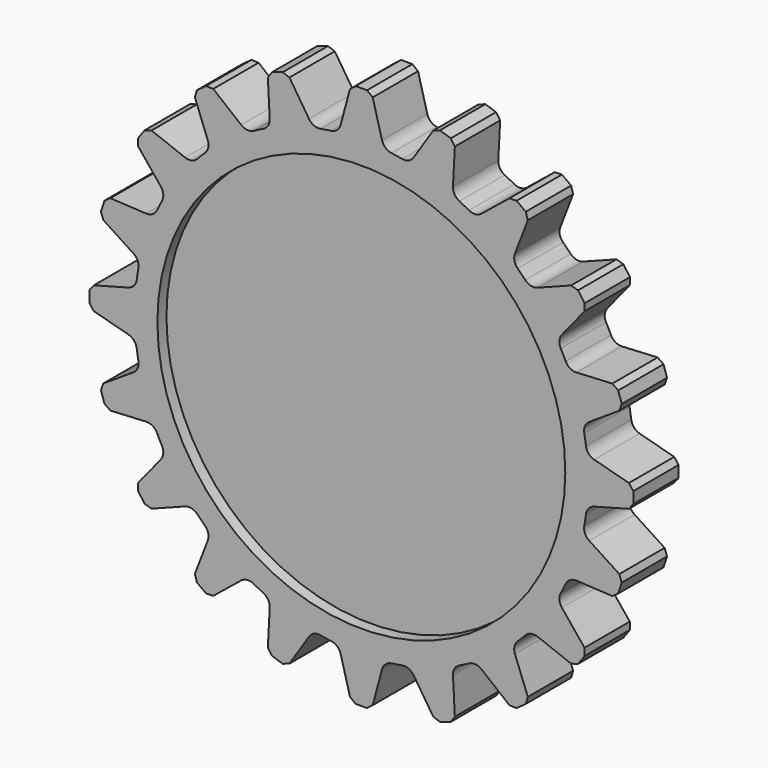
from build123d import *

# Parameters (mm, degrees)
F0_R            = 100
F1_DEPTH        = 25
F3_DEPTH        = 25
F3_COPIES_COUNT = 20
F4_SIZE         = 2
F5_R            = 5
F6_R            = 90
F7_DEPTH        = 5


# Not quite as in the source:
# - a pattern or mirror of a feature is missing from the dataset's text; its kind, count and spacing are read off the source's solid


with BuildPart() as f1:
    # F0 (on Front) → F1 (new body)
    with BuildSketch(Plane.XZ):
        Circle(F0_R)
    extrude(amount=F1_DEPTH)

    # F2 (on Front) → F3 (join)
    with BuildSketch(Plane.XZ):
        Polygon((4.5, 120), (-4.5, 120), (-9.9931095726, 99.4994359837), (9.9931095726, 99.4994359837), align=None)
    f3 = extrude(amount=F3_DEPTH)

    # F3_copies: F3 ×20 about axis
    f3_copies_axis = Axis((0, 0, 0), (0, 1, 0))
    for i in range(1, F3_COPIES_COUNT):
        add(f3.rotate(f3_copies_axis, i * 360 / F3_COPIES_COUNT))

    # F4
    f4_edges = [f1.edges().sort_by_distance(p)[0] for p in [
        (4.5, -12.5, 120),
        (-4.5, -12.5, 120),
        (-32.802285, -12.5, 115.517358),
        (115.517358, -12.5, 32.802285),
        (120, -12.5, 4.5),
        (120, -12.5, -4.5),
        (115.517358, -12.5, -32.802285),
        (112.736205, -12.5, -41.361794),
        (99.727073, -12.5, -66.893654),
        (94.437006, -12.5, -74.174807),
        (74.174807, -12.5, -94.437006),
        (66.893654, -12.5, -99.727073),
        (41.361794, -12.5, -112.736205),
        (32.802285, -12.5, -115.517358),
        (4.5, -12.5, -120),
        (-4.5, -12.5, -120),
        (-32.802285, -12.5, -115.517358),
        (-41.361794, -12.5, -112.736205),
        (-66.893654, -12.5, -99.727073),
        (-74.174807, -12.5, -94.437006),
        (-94.437006, -12.5, -74.174807),
        (-99.727073, -12.5, -66.893654),
        (-112.736205, -12.5, -41.361794),
        (-115.517358, -12.5, -32.802285),
        (-120, -12.5, -4.5),
        (-120, -12.5, 4.5),
        (-115.517358, -12.5, 32.802285),
        (-112.736205, -12.5, 41.361794),
        (-99.727073, -12.5, 66.893654),
        (-94.437006, -12.5, 74.174807),
        (-74.174807, -12.5, 94.437006),
        (-66.893654, -12.5, 99.727073),
        (32.802285, -12.5, 115.517358),
        (41.361794, -12.5, 112.736205),
        (66.893654, -12.5, 99.727073),
        (74.174807, -12.5, 94.437006),
        (94.437006, -12.5, 74.174807),
        (99.727073, -12.5, 66.893654),
        (112.736205, -12.5, 41.361794),
        (-41.361794, -12.5, 112.736205),
    ]]
    chamfer(f4_edges, length=F4_SIZE)

    # F5
    f5_edges = [f1.edges().sort_by_distance(p)[0] for p in [
        (9.99311, -12.5, 99.499436),
        (-9.99311, -12.5, 99.499436),
        (97.717628, -12.5, 21.243005),
        (99.499436, -12.5, 9.99311),
        (91.541546, -12.5, 40.251029),
        (86.370537, -12.5, 50.399706),
        (99.499436, -12.5, -9.99311),
        (97.717628, -12.5, -21.243005),
        (74.622932, -12.5, 66.568897),
        (66.568897, -12.5, 74.622932),
        (91.541546, -12.5, -40.251029),
        (86.370537, -12.5, -50.399706),
        (50.399706, -12.5, 86.370537),
        (40.251029, -12.5, 91.541546),
        (74.622932, -12.5, -66.568897),
        (66.568897, -12.5, -74.622932),
        (21.243005, -12.5, 97.717628),
        (50.399706, -12.5, -86.370537),
        (40.251029, -12.5, -91.541546),
        (-21.243005, -12.5, 97.717628),
        (21.243005, -12.5, -97.717628),
        (9.99311, -12.5, -99.499436),
        (-40.251029, -12.5, 91.541546),
        (-50.399706, -12.5, 86.370537),
        (-9.99311, -12.5, -99.499436),
        (-21.243005, -12.5, -97.717628),
        (-66.568897, -12.5, 74.622932),
        (-74.622932, -12.5, 66.568897),
        (-40.251029, -12.5, -91.541546),
        (-50.399706, -12.5, -86.370537),
        (-86.370537, -12.5, 50.399706),
        (-91.541546, -12.5, 40.251029),
        (-66.568897, -12.5, -74.622932),
        (-74.622932, -12.5, -66.568897),
        (-97.717628, -12.5, 21.243005),
        (-99.499436, -12.5, 9.99311),
        (-86.370537, -12.5, -50.399706),
        (-91.541546, -12.5, -40.251029),
        (-99.499436, -12.5, -9.99311),
        (-97.717628, -12.5, -21.243005),
    ]]
    fillet(f5_edges, radius=F5_R)

    # F6 (on face) → F7 (cut)
    with BuildSketch(Plane.XZ.offset(25)):
        Circle(F6_R)
    extrude(amount=-F7_DEPTH, mode=Mode.SUBTRACT)


solid = f1.part
